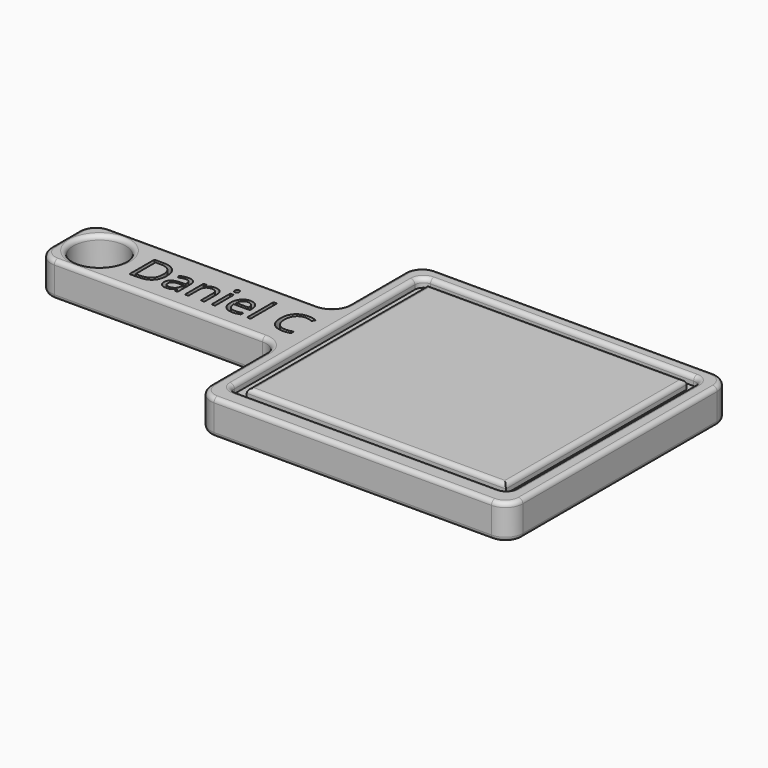
from build123d import *

# Parameters (mm, degrees)
F0_W         = 177.8
F0_H         = 50.8
F1_DEPTH     = 25.4
F2_R         = 19.05
F3_DEPTH     = 25.4
F4_W         = 205.3855772556
F4_H         = 177.8
F4_W_2       = 189.6664745388
F4_H_2       = 165.5154631916
F5_DEPTH     = 6.35
F6_R         = 6.35
F7_R         = 12.7
F8_R         = 3.17499
F9_TEXT_SIZE = 31.8518195388
F10_DEPTH    = 6.35


# Not quite as in the source:
# - a fillet or chamfer is up to 0.001 mm smaller than in the source, because OpenCascade refuses the exact size
# - Text() gives the source's letters only with a copy of the font that has no kerning and outlines rounded to 1/6400 em; it was checked with that copy


with BuildPart() as f1:
    # F0 (on Top) → F1 (new body)
    with BuildSketch(Plane.XY):
        with Locations((-88.9, 101.6)):
            Rectangle(F0_W, F0_H)
        Polygon((0, 76.2), (0, 0), (228.6, 0), (228.6, 203.2), (0, 203.2), (0, 127), align=None)
    extrude(amount=F1_DEPTH)

    # F2 (on face) → F3 (cut)
    with BuildSketch(Plane.XY.offset(25.4)):
        with Locations((-152.4, 101.6)):
            Circle(F2_R)
    extrude(amount=-F3_DEPTH, mode=Mode.SUBTRACT)

    # F4 (on face) → F5 (cut)
    with BuildSketch(Plane.XY.offset(25.4)):
        with Locations((113.6867667083, 103.4009051509)):
            Rectangle(F4_W, F4_H)
        with Locations((114.7111153369, 103.7431691168)):
            Rectangle(F4_W_2, F4_H_2, mode=Mode.SUBTRACT)
    extrude(amount=-F5_DEPTH, mode=Mode.SUBTRACT)

    # F6
    f6_edges = [f1.edges().sort_by_distance(p)[0] for p in [
        (10.993978, 192.300905, 22.225),
        (10.993978, 14.500905, 22.225),
        (216.379555, 192.300905, 22.225),
        (216.379555, 14.500905, 22.225),
    ]]
    fillet(f6_edges, radius=F6_R)

    # F7
    f7_edges = [f1.edges().sort_by_distance(p)[0] for p in [
        (0, 203.2, 12.7),
        (-177.8, 127, 12.7),
        (-177.8, 76.2, 12.7),
        (0, 0, 12.7),
        (228.6, 0, 12.7),
        (228.6, 203.2, 12.7),
        (0, 127, 12.7),
        (0, 76.2, 12.7),
    ]]
    fillet(f7_edges, radius=F7_R)

    # F8 (radius 3.175 in the source; OpenCascade refuses exactly that, so slightly less here)
    f8_edges = [f1.edges().sort_by_distance(p)[0] for p in [
        (19.877878, 103.743169, 25.4),
        (114.711115, 186.500901, 25.4),
        (209.544353, 103.743169, 25.4),
        (114.711115, 20.985438, 25.4),
        (-88.9, 76.2, 25.4),
        (-174.080256, 79.919744, 25.4),
        (-3.719744, 72.480256, 25.4),
        (-177.8, 101.6, 25.4),
        (0, 38.1, 25.4),
        (-174.080256, 123.280256, 25.4),
        (3.719744, 3.719744, 25.4),
        (-88.9, 127, 25.4),
        (114.3, 0, 25.4),
        (-3.719744, 130.719744, 25.4),
        (224.880256, 3.719744, 25.4),
        (0, 165.1, 25.4),
        (228.6, 101.6, 25.4),
        (3.719744, 199.480256, 25.4),
        (224.880256, 199.480256, 25.4),
        (114.3, 203.2, 25.4),
        (113.686767, 14.500905, 25.4),
        (12.85385, 16.360777, 25.4),
        (214.519683, 16.360777, 25.4),
        (10.993978, 103.400905, 25.4),
        (216.379555, 103.400905, 25.4),
        (12.85385, 190.441033, 25.4),
        (214.519683, 190.441033, 25.4),
        (113.686767, 192.300905, 25.4),
        (-171.45, 101.6, 25.4),
        (-88.9, 76.2, 0),
        (-174.080256, 79.919744, 0),
        (-3.719744, 72.480256, 0),
        (-177.8, 101.6, 0),
        (0, 38.1, 0),
        (-174.080256, 123.280256, 0),
        (3.719744, 3.719744, 0),
        (-88.9, 127, 0),
        (114.3, 0, 0),
        (-3.719744, 130.719744, 0),
        (224.880256, 3.719744, 0),
        (0, 165.1, 0),
        (228.6, 101.6, 0),
        (3.719744, 199.480256, 0),
        (224.880256, 199.480256, 0),
        (114.3, 203.2, 0),
        (-171.45, 101.6, 0),
    ]]
    fillet(f8_edges, radius=F8_R)

    # F9 (on face) → F10 (cut)
    with BuildSketch(Plane.XY.offset(25.4)):
        with Locations((-123.9583233206, 89.6265879273)):
            Text('Daniel C', F9_TEXT_SIZE, font='Open Sans', text_align=(TextAlign.LEFT, TextAlign.BOTTOM))
    extrude(amount=-F10_DEPTH, mode=Mode.SUBTRACT)


solid = f1.part
